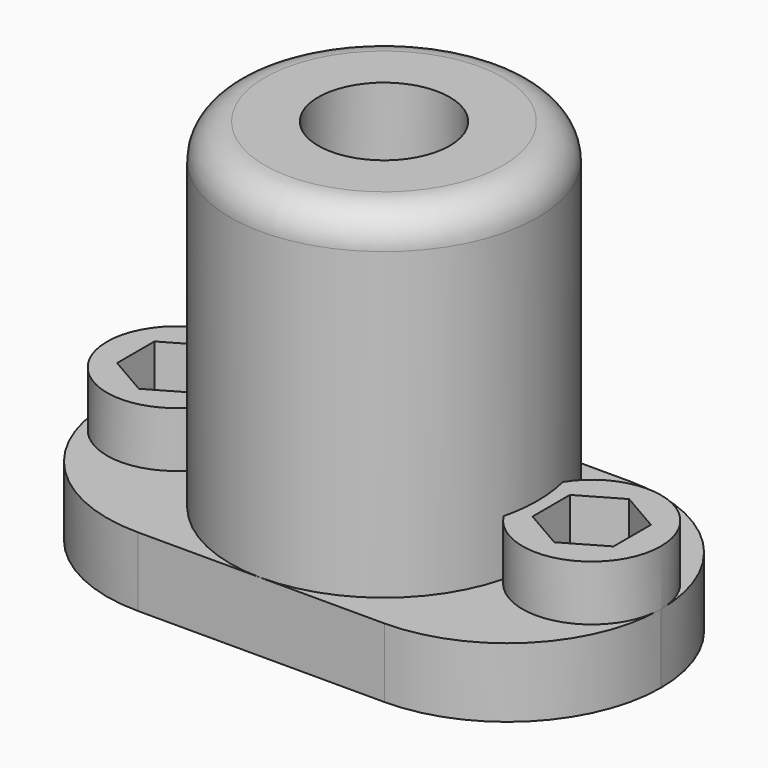
from build123d import *

# Parameters (mm, degrees)
F0_W     = 40
F0_H     = 22.2
F0_R     = 2.125
F0_R_2   = 7.825
F1_DEPTH = 5
F2_R     = 11.1
F2_R_2   = 7.825
F3_DEPTH = 19.5
F4_R     = 11.1
F4_R_2   = 4.75
F5_DEPTH = 5
F6_R     = 11.09999
F7_R     = 2.5
F8_R     = 5
F9_DEPTH = 4


# Not quite as in the source:
# - a fillet or chamfer is up to 0.001 mm smaller than in the source, because OpenCascade refuses the exact size


with BuildPart() as f1:
    # F0 (on Top) → F1 (new body)
    with BuildSketch(Plane.XY):
        Rectangle(F0_W, F0_H)
        with Locations((-15, 0)):
            Circle(F0_R, mode=Mode.SUBTRACT)
        Circle(F0_R_2, mode=Mode.SUBTRACT)
        with Locations((15, 0)):
            Circle(F0_R, mode=Mode.SUBTRACT)
    extrude(amount=F1_DEPTH)

    # F2 (on face) → F3 (join)
    with BuildSketch(Plane.XY.offset(5)):
        Circle(F2_R)
        Circle(F2_R_2, mode=Mode.SUBTRACT)
    extrude(amount=F3_DEPTH)

    # F4 (on face) → F5 (join)
    with BuildSketch(Plane.XY.offset(24.5)):
        Circle(F4_R)
        Circle(F4_R_2, mode=Mode.SUBTRACT)
    extrude(amount=F5_DEPTH)

    # F6 (radius 11.1 in the source; OpenCascade refuses exactly that, so slightly less here)
    f6_edges = [f1.edges().sort_by_distance(p)[0] for p in [
        (-20, 11.1, 2.5),
        (-20, -11.1, 2.5),
        (20, -11.1, 2.5),
        (20, 11.1, 2.5),
    ]]
    fillet(f6_edges, radius=F6_R)

    # F7
    f7_edges = [f1.edges().sort_by_distance(p)[0] for p in [
        (-11.1, 0, 29.5),
    ]]
    fillet(f7_edges, radius=F7_R)

    # F8 (on face) → F9 (join)
    with BuildSketch(Plane.XY.offset(5)):
        with Locations((-15, 0)):
            Circle(F8_R)
        Polygon((-15, 3.3774990748), (-12.075, 1.6887495374), (-12.075, -1.6887495374), (-15, -3.3774990748), (-17.925, -1.6887495374), (-17.925, 1.6887495374), align=None, mode=Mode.SUBTRACT)
        with Locations((15, 0)):
            Circle(F8_R)
        Polygon((12.075, -1.6887495374), (12.075, 1.6887495374), (15, 3.3774990748), (17.925, 1.6887495374), (17.925, -1.6887495374), (15, -3.3774990748), align=None, mode=Mode.SUBTRACT)
    extrude(amount=F9_DEPTH)


solid = f1.part
